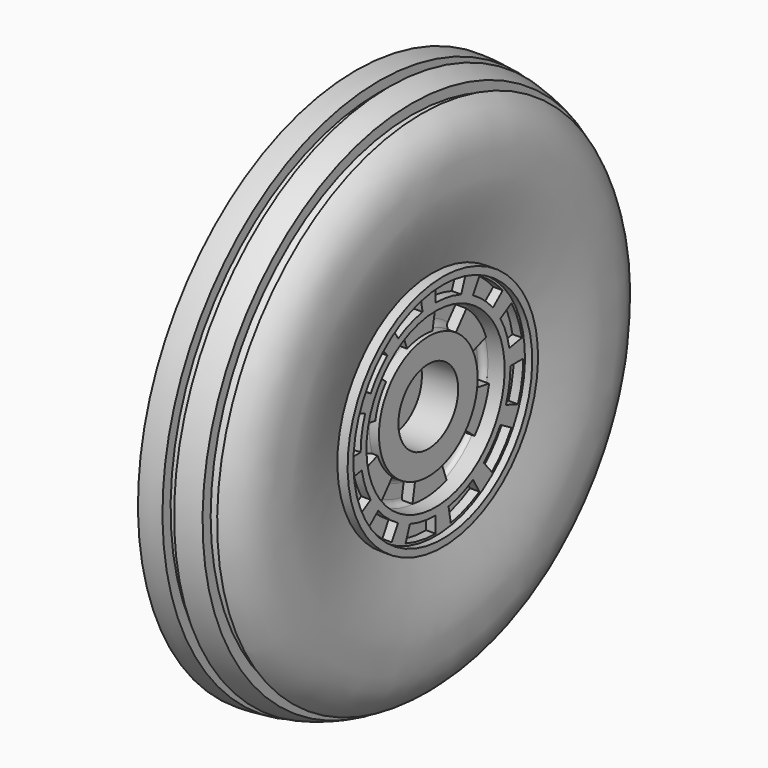
from build123d import *

# Parameters (mm, degrees)
F2_W            = 0.2
F2_H            = 0.22
F3_ANGLE        = 20
F3_COPIES_COUNT = 12
F5_DEPTH        = 0.15


# Not quite as in the source:
# - a pattern or mirror of a feature is missing from the dataset's text; its kind, count and spacing are read off the source's solid


with BuildPart() as f1:
    # F0 (on Front) → F1 (revolve)
    with BuildSketch(Plane.XZ):
        with BuildLine():
            Line((1, 0.85), (0.87, 0.85))
            ThreePointArc((0.87, 0.85), (0.8134314575, 0.8734314575), (0.79, 0.93))
            Line((0.79, 0.93), (0.79, 1.11))
            ThreePointArc((0.79, 1.11), (0.8134314575, 1.1665685425), (0.87, 1.19))
            Line((0.87, 1.19), (1.1, 1.19))
            Line((1.1, 1.19), (1.1, 1.54))
            Line((1.1, 1.54), (1.2, 1.54))
            Line((1.2, 1.54), (1.2, 1.64))
            Line((1.2, 1.64), (1.12, 1.64))
            Line((1.12, 1.64), (1.0590550792, 1.64))
            add(Edge.make_bspline(
                [(1.0590550792, 1.64), (1.25, 2.3421209771), (1.2635455001, 2.685534462), (1.2259744013, 3.2558219262), (0.9930693577, 3.4693235058), (0.91, 3.5233867214)],
                knots=[0, 0, 0, 0, 0.3714125336, 0.6273384476, 0.7316891336, 0.7316891336, 0.7316891336, 0.7316891336], degree=3))
            Line((0.91, 3.5233867214), (0.91, 3.3833867214))
            Line((0.91, 3.3833867214), (0.77, 3.4602341654))
            Line((0.77, 3.4602341654), (0.77, 3.6002341654))
            add(Edge.make_bspline(
                [(0.77, 3.6002341654), (0.6784642229, 3.6425426702), (0.5744947558, 3.6771881754), (0.46, 3.7024604996)],
                knots=[0.7852748547, 0.7852748547, 0.7852748547, 0.7852748547, 0.8822719118, 0.8822719118, 0.8822719118, 0.8822719118], degree=3))
            Line((0.46, 3.7024604996), (0.46, 3.5624604996))
            Line((0.46, 3.5624604996), (0.32, 3.5878456739))
            Line((0.32, 3.5878456739), (0.32, 3.7278456739))
            add(Edge.make_bspline(
                [(0.32, 3.7278456739), (0.2195553432, 3.7423008552), (0.1125378698, 3.75), (0, 3.75)],
                knots=[0.9204576606, 0.9204576606, 0.9204576606, 0.9204576606, 1, 1, 1, 1], degree=3))
            Line((0, 3.75), (0, 2.75))
            Line((0, 2.75), (0.2, 2.75))
            Line((0.2, 2.75), (0.2, 2.55))
            Line((0.2, 2.55), (0.5, 2.55))
            Line((0.5, 2.55), (0.5, 2.15))
            Line((0.5, 2.15), (0.02, 2.15))
            Line((0.02, 2.15), (0.02, 0))
            Line((0.02, 0), (0.5, 0))
            Line((0.5, 0), (0.5, 0.515))
            Line((0.5, 0.515), (1, 0.515))
            Line((1, 0.515), (1, 0.85))
        make_face()
    revolve(axis=Axis((1.052, 0, 0), (1, 0, 0)))

    # F2 (on Front) → F3 (revolve, cut)
    with BuildSketch(Plane.XZ):
        with Locations((1.07, 1.4)):
            Rectangle(F2_W, F2_H)
    f3 = revolve(axis=Axis((1.36, 0, 0), (-1, 0, 0)), revolution_arc=F3_ANGLE, mode=Mode.SUBTRACT)

    # F3_copies: F3 ×12 about axis
    f3_copies_axis = Axis((0, 0, 0), (1, 0, 0))
    for i in range(1, F3_COPIES_COUNT):
        add(f3.rotate(f3_copies_axis, i * 360 / F3_COPIES_COUNT), mode=Mode.SUBTRACT)

    # F4 (on face) → F5 (join)
    with BuildSketch(Plane.YZ.offset(0.79)):
        with BuildLine():
            Line((-0.3895609432, 1.0703098951), (-0.2696546218, 0.7408699845))
            ThreePointArc((-0.2696546218, 0.7408699845), (-0.0687151015, 0.7854172037), (0.1369072395, 0.7764395384))
            Line((0.1369072395, 0.7764395384), (0.1977852744, 1.1216960307))
            ThreePointArc((0.1977852744, 1.1216960307), (-0.099270391, 1.1346657611), (-0.3895609432, 1.0703098951))
        make_face()
        with BuildLine():
            Line((-1.1216960307, 0.1977852744), (-0.7764395384, 0.1369072395))
            ThreePointArc((-0.7764395384, 0.1369072395), (-0.7145488017, 0.3331995784), (-0.603962745, 0.5067849166))
            Line((-0.603962745, 0.5067849166), (-0.8725246207, 0.7321350874))
            ThreePointArc((-0.8725246207, 0.7321350874), (-1.0322845694, 0.4813622001), (-1.1216960307, 0.1977852744))
        make_face()
        with BuildLine():
            Line((-0.7321350874, -0.8725246207), (-0.5067849166, -0.603962745))
            ThreePointArc((-0.5067849166, -0.603962745), (-0.6458337002, -0.4522176253), (-0.7408699845, -0.2696546218))
            Line((-0.7408699845, -0.2696546218), (-1.0703098951, -0.3895609432))
            ThreePointArc((-1.0703098951, -0.3895609432), (-0.9330141784, -0.653303561), (-0.7321350874, -0.8725246207))
        make_face()
        with BuildLine():
            Line((0.3895609432, -1.0703098951), (0.2696546218, -0.7408699845))
            ThreePointArc((0.2696546218, -0.7408699845), (0.0687151015, -0.7854172037), (-0.1369072395, -0.7764395384))
            Line((-0.1369072395, -0.7764395384), (-0.1977852744, -1.1216960307))
            ThreePointArc((-0.1977852744, -1.1216960307), (0.099270391, -1.1346657611), (0.3895609432, -1.0703098951))
        make_face()
        with BuildLine():
            Line((1.1216960307, -0.1977852744), (0.7764395384, -0.1369072395))
            ThreePointArc((0.7764395384, -0.1369072395), (0.7145488017, -0.3331995784), (0.603962745, -0.5067849166))
            Line((0.603962745, -0.5067849166), (0.8725246207, -0.7321350874))
            ThreePointArc((0.8725246207, -0.7321350874), (1.0322845694, -0.4813622001), (1.1216960307, -0.1977852744))
        make_face()
        with BuildLine():
            Line((0.7321350874, 0.8725246207), (0.5067849166, 0.603962745))
            ThreePointArc((0.5067849166, 0.603962745), (0.6458337002, 0.4522176253), (0.7408699845, 0.2696546218))
            Line((0.7408699845, 0.2696546218), (1.0703098951, 0.3895609432))
            ThreePointArc((1.0703098951, 0.3895609432), (0.9330141784, 0.653303561), (0.7321350874, 0.8725246207))
        make_face()
    extrude(amount=F5_DEPTH)


solid = f1.part
